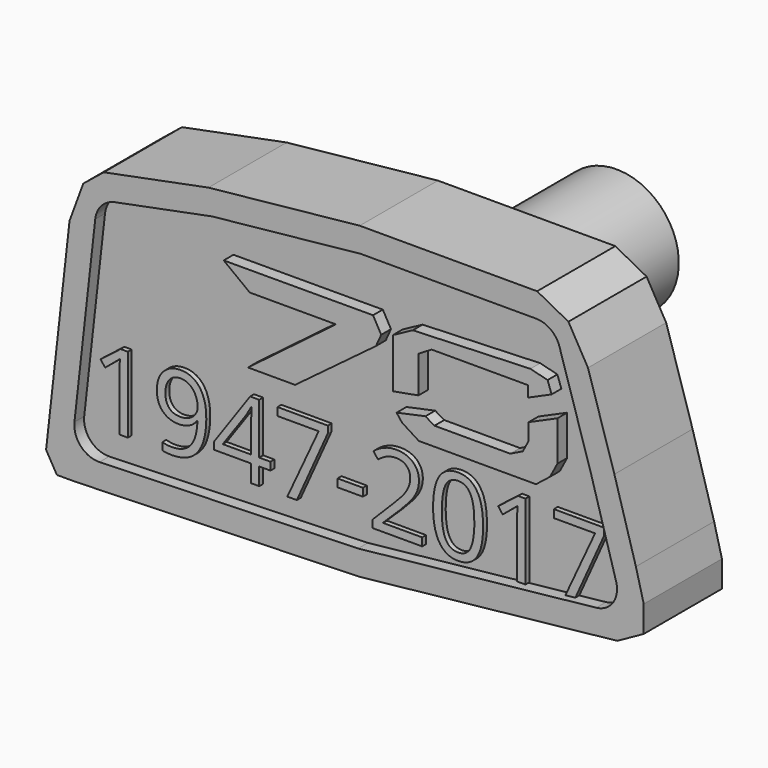
from build123d import *

# Parameters (mm, degrees)
F1_DEPTH     = 4
F3_DEPTH     = 0.5
F5_DEPTH     = 0.5
F6_TEXT_SIZE = 4.3365475398
F7_DEPTH     = 0.2
F8_R         = 2.5443255032
F9_DEPTH     = 10
F10_SCALE    = 3


# Not quite as in the source:
# - Text() gives the source's letters only with a copy of the font that has no kerning and outlines rounded to 1/6400 em; it was checked with that copy


with BuildPart() as f1:
    # F0 (on Front) → F1 (new body)
    with BuildSketch(Plane.XZ):
        Polygon((-11.8744745851, 3.1425706111), (-12.8351859748, -5.423778668), (-12.3948603868, -6.1843423173), (-11.6342967376, -6.1843423173), (0, -5.8240755461), (10.5421403423, -4.70324466), (11.6229411215, -4.1027995758), (11.6229411215, -3.0219985638), (11.3027030602, -1.781078754), (10.4220509529, 1.2611761922), (9.3412501737, 4.7437576577), (8.5406564176, 6.1447960325), (7.2597074322, 6.8252999336), (4.8178974539, 6.8252999336), (0, 6.8252999336), (-6.1902618036, 6.1848247424), (-10.473436676, 5.344202742), (-11.3140586764, 4.6636979096), align=None)
    extrude(amount=F1_DEPTH)

    # F2 (on face) → F3 (cut)
    with BuildSketch(Plane.XZ.offset(4)):
        with BuildLine():
            Line((-10.6492737519, -5.1533608391), (-0.0684332678, -4.8257153162))
            Line((-0.0684332678, -4.8257153162), (9.6850504296, -3.7887336958))
            ThreePointArc((9.6850504296, -3.7887336958), (10.370661573, -3.3753471671), (10.4941703959, -2.5843372856))
            Line((10.4941703959, -2.5843372856), (9.4641489068, 0.9739213548))
            Line((9.4641489068, 0.9739213548), (8.176907986, 5.121699057))
            ThreePointArc((8.176907986, 5.121699057), (7.8149714953, 5.6304083497), (7.2218438208, 5.8252999336))
            Line((7.2218438208, 5.8252999336), (0.0515947672, 5.8252999336))
            Line((0.0515947672, 5.8252999336), (-6.042206043, 5.1948050752))
            Line((-6.042206043, 5.1948050752), (-10.0220148109, 4.4137221385))
            ThreePointArc((-10.0220148109, 4.4137221385), (-10.564962331, 4.1099291477), (-10.8231973918, 3.5438930674))
            Line((-10.8231973918, 3.5438930674), (-11.6739947997, -4.0423891812))
            ThreePointArc((-11.6739947997, -4.0423891812), (-11.4152891584, -4.8318373215), (-10.6492737519, -5.1533608391))
        make_face()
    extrude(amount=-F3_DEPTH, mode=Mode.SUBTRACT)

    # F4 (on face) → F5 (join)
    with BuildSketch(Plane.XZ.offset(3.5)):
        Polygon((0.5453656777, 3.7770913914), (-5.5664332416, 3.7653651983), (-4.4985357672, 2.9545540456), (-0.9743764992, 2.9545540456), (-4.572017584, 0.2306257957), (-2.6440734509, 0.2306257957), (0.6643746165, 2.7060110588), (0.8785904502, 3.1820468139), align=None)
        Polygon((6.9862916134, 3.9416956715), (2.1727116553, 3.7653651983), (1.3546261471, 3.3248576801), (1.3546261471, 2.3013809696), (1.3546261471, 1.3017059537), (2.4019044358, 1.4921203256), (2.4019044358, 2.9916325584), (2.9404995195, 3.3207740635), (6.8847797168, 3.3207740635), (6.8847797168, 2.8711734707), (7.8525133431, 3.3010558691), (7.6887366662, 3.7653651983), align=None)
        Polygon((2.6880460791, 0.8339232882), (1.5099180164, 0.5814672331), (1.728713396, 0.2953505027), (2.4187597446, -0.1422400819), (7.2154244408, -0.1422400819), (7.7876579016, 0.3121807822), (8.090605028, 0.8844145341), (8.090605028, 2.5169635192), (6.9124768488, 1.9952210132), (6.9124768488, 1.3220049441), (6.6768517718, 0.8675841382), (6.155109033, 0.6151280832), (3.0583150219, 0.6151280832), align=None)
    extrude(amount=F5_DEPTH)

    # F6 (on face) → F7 (join)
    with BuildSketch(Plane.XZ.offset(3.5)):
        with Locations((-11.2441002857, -4.0975871379)):
            Text('1947-2017', F6_TEXT_SIZE, font='Open Sans', text_align=(TextAlign.LEFT, TextAlign.BOTTOM))
    extrude(amount=F7_DEPTH)

    # F8 (on face) → F9 (join)
    with BuildSketch(Plane(origin=(0, 0, 0), x_dir=(-1, 0, 0), z_dir=(0, 1, 0))):
        with Locations((0.6861825241, 0.399703189)):
            Circle(F8_R)
    extrude(amount=F9_DEPTH)


with BuildPart() as f1_1:
    # F10: moved
    add(f1.part.scale(F10_SCALE))


solid = f1_1.part
